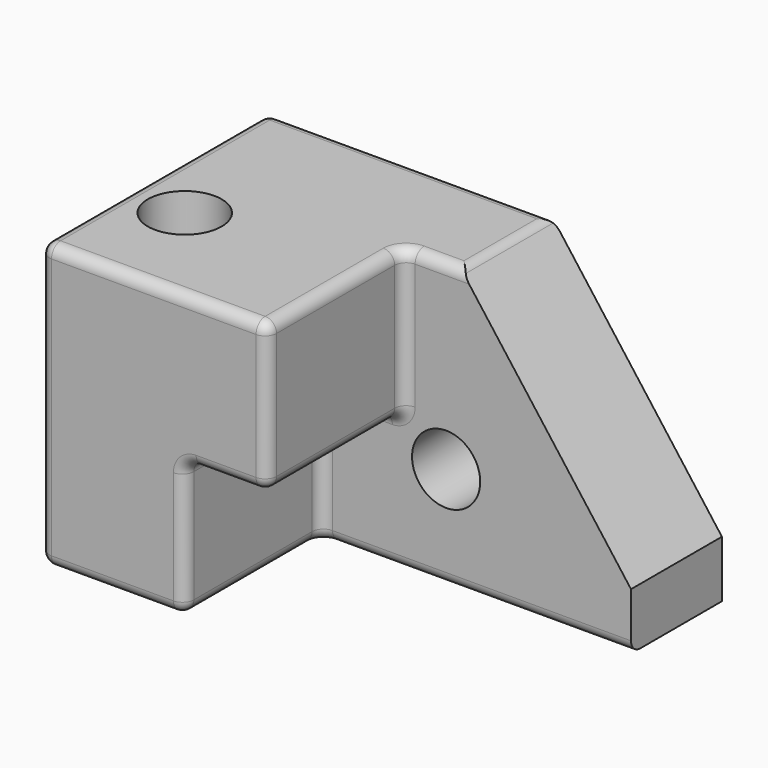
from build123d import *

# Parameters (mm, degrees)
F0_W     = 203.2
F0_H     = 127
F1_DEPTH = 127
F3_DEPTH = 76.2
F4_SIZE2 = 101.6
F4_SIZE  = 76.2
F5_R     = 5.08
F6_R     = 15.24
F7_DEPTH = 50.8
F8_R     = 16.51
F9_DEPTH = 127


with BuildPart() as f1:
    # F0 (on Front) → F1 (new body)
    with BuildSketch(Plane.XZ):
        with Locations((0, 2.9180156587)):
            Rectangle(F0_W, F0_H)
    extrude(amount=F1_DEPTH)

    # F2 (on face) → F3 (cut)
    with BuildSketch(Plane.XZ.offset(127)):
        Polygon((-36.9453281164, 0), (-36.9453281164, -60.5819843413), (101.6, -60.5819843413), (101.6, 66.4180156587), (0, 66.4180156587), (0, 0), align=None)
    extrude(amount=-F3_DEPTH, mode=Mode.SUBTRACT)

    # F4
    f4_edges = [f1.edges().sort_by_distance(p)[0] for p in [
        (101.6, -25.4, 66.418016),
    ]]
    f4_side = f1.faces().sort_by_distance((-21.771429, -52.614286, 66.418016))[0]
    chamfer(f4_edges, length=F4_SIZE, length2=F4_SIZE2, reference=f4_side)

    # F5
    f5_edges = [f1.edges().sort_by_distance(p)[0] for p in [
        (-38.1, 0, 66.418016),
        (25.4, -25.4, 66.418016),
        (-101.6, -63.5, 66.418016),
        (12.7, -50.8, 66.418016),
        (-50.8, -127, 66.418016),
        (0, -88.9, 66.418016),
        (0, -88.9, 0),
        (0, -127, 33.209008),
        (0, -50.8, 33.209008),
        (-69.272664, -127, -60.581984),
        (-101.6, -127, 2.918016),
        (-18.472664, -127, 0),
        (-36.945328, -127, -30.290992),
        (-36.945328, -88.9, 0),
        (-36.945328, -88.9, -60.581984),
        (-36.945328, -50.8, -30.290992),
        (-101.6, -63.5, -60.581984),
        (-101.6, 0, 2.918016),
        (32.327336, -50.8, -60.581984),
        (-18.472664, -50.8, 0),
    ]]
    fillet(f5_edges, radius=F5_R)

    # F6 (on face) → F7 (cut, through all)
    with BuildSketch(Plane.XZ.offset(50.8)):
        with Locations((18.9346718836, -14.8619843413)):
            Circle(F6_R)
    extrude(amount=-F7_DEPTH, mode=Mode.SUBTRACT)

    # F8 (on face) → F9 (cut, through all)
    with BuildSketch(Plane.XY.offset(66.4180156587)):
        with Locations((-75.8790969849, -78.356936574)):
            Circle(F8_R)
    extrude(amount=-F9_DEPTH, mode=Mode.SUBTRACT)


solid = f1.part
